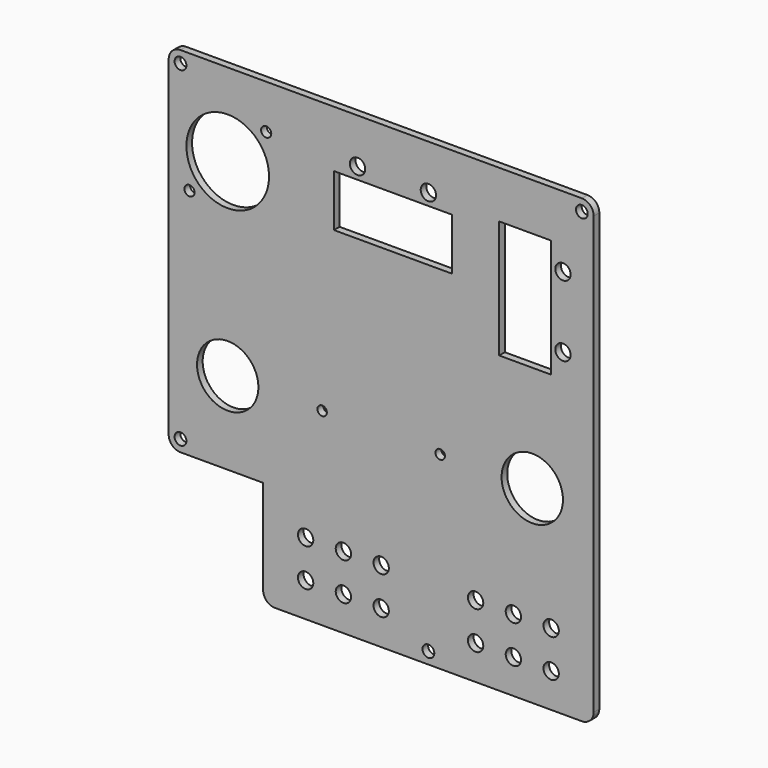
from build123d import *

# Parameters (mm, degrees)
F1_DEPTH = 3
F2_R     = 17.5
F2_R_2   = 13
F2_R_3   = 2
F2_W     = 22
F2_H     = 50
F2_W_2   = 50
F2_H_2   = 22
F3_DEPTH = 3
F4_R     = 2.5
F5_DEPTH = 3
F6_R     = 3.25
F7_DEPTH = 3
F8_R     = 3.25
F9_DEPTH = 3
F10_R    = 5


# Not quite as in the source:
# - a feature names something its author has since deleted; it is built from what else it names


with BuildPart() as f1:
    # F0 (on Front) → F1 (new body)
    with BuildSketch(Plane.XZ):
        Polygon((90, -75), (90, 75), (-90, 75), (-90, -75), (-50, -75), (-50, -120), (90, -120), align=None)
    extrude(amount=F1_DEPTH)

    # F2 (on face) → F3 (cut, through all)
    with BuildSketch(Plane.XZ.offset(3)):
        with Locations((-65, 40)):
            Circle(F2_R)
        with Locations((-65, -40)):
            Circle(F2_R_2)
        with BuildLine():
            ThreePointArc((-50.3238814883, 57.7090808748), (-50.2202795796, 54.7797204204), (-47.2909191252, 54.6761185117))
            ThreePointArc((-47.2909191252, 54.6761185117), (-48.7365440327, 56.2634559673), (-50.3238814883, 57.7090808748))
        make_face()
        with BuildLine():
            ThreePointArc((-50.3238814883, 57.7090808748), (-48.7365440327, 56.2634559673), (-47.2909191252, 54.6761185117))
            ThreePointArc((-47.2909191252, 54.6761185117), (-46.7439805879, 55.4075382028), (-46.55, 56.3))
            ThreePointArc((-46.55, 56.3), (-47.9479511984, 58.3141803792), (-50.3238814883, 57.7090808748))
        make_face()
        with BuildLine():
            ThreePointArc((-82.7125051724, 25.3280144317), (-82.7202795796, 22.2797204204), (-79.6719855683, 22.2874948276))
            ThreePointArc((-79.6719855683, 22.2874948276), (-81.2634559673, 23.7365440327), (-82.7125051724, 25.3280144317))
        make_face()
        with BuildLine():
            ThreePointArc((-82.7125051724, 25.3280144317), (-81.2634559673, 23.7365440327), (-79.6719855683, 22.2874948276))
            ThreePointArc((-79.6719855683, 22.2874948276), (-79.2115670708, 22.9822992687), (-79.05, 23.8))
            ThreePointArc((-79.05, 23.8), (-80.3721673239, 25.7842361403), (-82.7125051724, 25.3280144317))
        make_face()
        with Locations((-25, -40)):
            Circle(F2_R_3)
        with Locations((25, -40)):
            Circle(F2_R_3)
        with Locations((64, -40)):
            Circle(F2_R_2)
        with Locations((61, 30)):
            Rectangle(F2_W, F2_H)
        with Locations((5, 40)):
            Rectangle(F2_W_2, F2_H_2)
    extrude(amount=-F3_DEPTH, mode=Mode.SUBTRACT)

    # F4 (on face) → F5 (cut, through all)
    with BuildSketch(Plane.XZ.offset(3)):
        with Locations((-85, 70)):
            Circle(F4_R)
        with Locations((85, 70)):
            Circle(F4_R)
        with Locations((20, -115)):
            Circle(F4_R)
        with Locations((-85, -70)):
            Circle(F4_R)
    extrude(amount=-F5_DEPTH, mode=Mode.SUBTRACT)

    # F6 (on face) → F7 (cut, through all)
    with BuildSketch(Plane.XZ.offset(3)):
        with Locations((-32, -89.5)):
            Circle(F6_R)
        with Locations((-16, -89.5)):
            Circle(F6_R)
        with Locations((0, -89.5)):
            Circle(F6_R)
        with Locations((40, -89.5)):
            Circle(F6_R)
        with Locations((56, -89.5)):
            Circle(F6_R)
        with Locations((72, -89.5)):
            Circle(F6_R)
        with Locations((72, -105.5)):
            Circle(F6_R)
        with Locations((56, -105.5)):
            Circle(F6_R)
        with Locations((40, -105.5)):
            Circle(F6_R)
        with Locations((-32, -105.5)):
            Circle(F6_R)
        with Locations((-16, -105.5)):
            Circle(F6_R)
        with Locations((0, -105.5)):
            Circle(F6_R)
    extrude(amount=-F7_DEPTH, mode=Mode.SUBTRACT)

    # F8 (on face) → F9 (cut, through all)
    with BuildSketch(Plane.XZ.offset(3)):
        with Locations((-10, 56)):
            Circle(F8_R)
        with Locations((20, 56)):
            Circle(F8_R)
        with Locations((77, 15)):
            Circle(F8_R)
        with Locations((77, 45)):
            Circle(F8_R)
    extrude(amount=-F9_DEPTH, mode=Mode.SUBTRACT)

    # F10
    f10_edges = [f1.edges().sort_by_distance(p)[0] for p in [
        (90, -1.5, 75),
        (-90, -1.5, 75),
        (-90, -1.5, -75),
        (-50, -1.5, -120),
        (90, -1.5, -120),
    ]]
    fillet(f10_edges, radius=F10_R)


solid = f1.part
